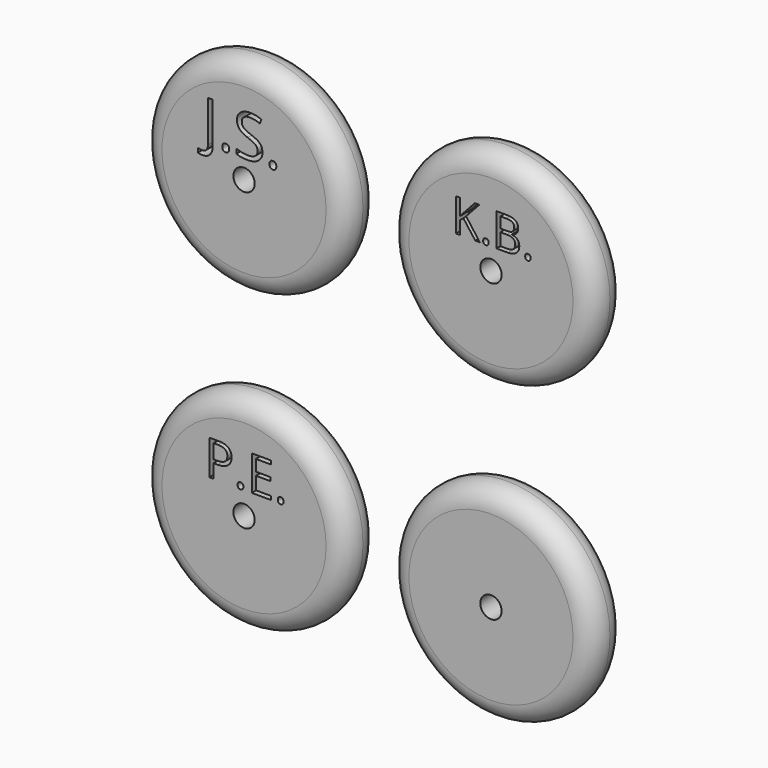
from build123d import *

# Parameters (mm, degrees)
F0_R           = 15.875
F1_DEPTH       = 6.35
F2_R           = 3.17499
F2_2_R         = 3.17499
F2_3_R         = 3.17499
F2_4_R         = 3.17499
F3_R           = 1.651
F4_DEPTH       = 25.4
F5_DEPTH       = 25.4
F6_DEPTH       = 25.4
F7_DEPTH       = 25.4
F8_TEXT_SIZE   = 8.9633877371
F8_TEXT_SIZE_2 = 7.1167148236
F8_TEXT_SIZE_3 = 7.555307678
F9_DEPTH       = 2.54
F10_DEPTH      = 2.54
F12_DEPTH      = 2.54
F11_TEXT_SIZE  = 3.4882623063
F13_DEPTH      = 0.508


# Not quite as in the source:
# - a fillet or chamfer is up to 0.001 mm smaller than in the source, because OpenCascade refuses the exact size
# - Text() gives the source's letters only with a copy of the font that has no kerning and outlines rounded to 1/6400 em; it was checked with that copy


with BuildPart() as f1:
    # F0 (on Front) → F1 (new body)
    with BuildSketch(Plane.XZ):
        with Locations((-57.9834368664, 37.8684985699)):
            Circle(F0_R)
    extrude(amount=F1_DEPTH)

    # F2#3 (radius 3.175 in the source; OpenCascade refuses exactly that, so slightly less here)
    f2_3_edges = [f1.edges().sort_by_distance(p)[0] for p in [
        (-73.858437, 0, 37.868499),
        (-73.858437, -6.35, 37.868499),
    ]]
    fillet(f2_3_edges, radius=F2_3_R)

    # F3 (on face) → F4 (cut)
    with BuildSketch(Plane.XZ.offset(6.35)):
        with Locations((-57.9834368664, 37.8684985699)):
            Circle(F3_R)
    extrude(amount=-F4_DEPTH, mode=Mode.SUBTRACT)


with BuildPart() as f1b:
    # F0 (on Front) → F1, piece 2 (new body)
    with BuildSketch(Plane.XZ):
        with Locations((-57.9834368664, -7.9332944006)):
            Circle(F0_R)
    extrude(amount=F1_DEPTH)

    # F2#4 (radius 3.175 in the source; OpenCascade refuses exactly that, so slightly less here)
    f2_4_edges = [f1b.edges().sort_by_distance(p)[0] for p in [
        (-73.858437, 0, -7.933294),
        (-73.858437, -6.35, -7.933294),
    ]]
    fillet(f2_4_edges, radius=F2_4_R)

    # F3 (on face) → F6 (cut)
    with BuildSketch(Plane.XZ.offset(6.35)):
        with Locations((-57.9834368664, -7.9332944006)):
            Circle(F3_R)
    extrude(amount=-F6_DEPTH, mode=Mode.SUBTRACT)


with BuildPart() as f1c:
    # F0 (on Front) → F1, piece 3 (new body)
    with BuildSketch(Plane.XZ):
        with Locations((-19.7645071894, -7.9332944006)):
            Circle(F0_R)
    extrude(amount=F1_DEPTH)

    # F2 (radius 3.175 in the source; OpenCascade refuses exactly that, so slightly less here)
    f2_edges = [f1c.edges().sort_by_distance(p)[0] for p in [
        (-35.639507, 0, -7.933294),
        (-35.639507, -6.35, -7.933294),
    ]]
    fillet(f2_edges, radius=F2_R)

    # F3 (on face) → F7 (cut)
    with BuildSketch(Plane.XZ.offset(6.35)):
        with Locations((-19.7645071894, -7.9332944006)):
            Circle(F3_R)
    extrude(amount=-F7_DEPTH, mode=Mode.SUBTRACT)


with BuildPart() as f1d:
    # F0 (on Front) → F1, piece 4 (new body)
    with BuildSketch(Plane.XZ):
        with Locations((-19.7645071894, 37.8684985699)):
            Circle(F0_R)
    extrude(amount=F1_DEPTH)

    # F2#2 (radius 3.175 in the source; OpenCascade refuses exactly that, so slightly less here)
    f2_2_edges = [f1d.edges().sort_by_distance(p)[0] for p in [
        (-35.639507, 0, 37.868499),
        (-35.639507, -6.35, 37.868499),
    ]]
    fillet(f2_2_edges, radius=F2_2_R)

    # F3 (on face) → F5 (cut)
    with BuildSketch(Plane.XZ.offset(6.35)):
        with Locations((-19.7645071894, 37.8684985699)):
            Circle(F3_R)
    extrude(amount=-F5_DEPTH, mode=Mode.SUBTRACT)


with BuildPart() as f9_tool:
    # F8 (on face) → F9 (new body)
    with BuildSketch(Plane.XZ.offset(6.35)):
        with Locations((-64.4037676054, 40.8216691305)):
            Text('J.S.', F8_TEXT_SIZE, font='Open Sans', text_align=(TextAlign.LEFT, TextAlign.BOTTOM))
        with Locations((-25.8644149952, 41.2169232358)):
            Text('K.B.', F8_TEXT_SIZE_2, font='Open Sans', text_align=(TextAlign.LEFT, TextAlign.BOTTOM))
        with Locations((-64.0788827856, -4.4081961426)):
            Text('P.E.', F8_TEXT_SIZE_3, font='Open Sans', text_align=(TextAlign.LEFT, TextAlign.BOTTOM))
    extrude(amount=-F9_DEPTH)


with BuildPart() as f1_1:
    add(f1.part)

    # F9: cut by f9_tool
    add(f9_tool.part, mode=Mode.SUBTRACT)

    # F8 (on face) → F10 (cut)
    with BuildSketch(Plane.XZ.offset(6.35)):
        with Locations((-64.4037676054, 40.8216691305)):
            Text('J.S.', F8_TEXT_SIZE, font='Open Sans', text_align=(TextAlign.LEFT, TextAlign.BOTTOM))
        with Locations((-25.8644149952, 41.2169232358)):
            Text('K.B.', F8_TEXT_SIZE_2, font='Open Sans', text_align=(TextAlign.LEFT, TextAlign.BOTTOM))
        with Locations((-64.0788827856, -4.4081961426)):
            Text('P.E.', F8_TEXT_SIZE_3, font='Open Sans', text_align=(TextAlign.LEFT, TextAlign.BOTTOM))
    extrude(amount=-F10_DEPTH, mode=Mode.SUBTRACT)

    # F8 (on face) → F12 (cut)
    with BuildSketch(Plane.XZ.offset(6.35)):
        with Locations((-64.4037676054, 40.8216691305)):
            Text('J.S.', F8_TEXT_SIZE, font='Open Sans', text_align=(TextAlign.LEFT, TextAlign.BOTTOM))
        with Locations((-25.8644149952, 41.2169232358)):
            Text('K.B.', F8_TEXT_SIZE_2, font='Open Sans', text_align=(TextAlign.LEFT, TextAlign.BOTTOM))
        with Locations((-64.0788827856, -4.4081961426)):
            Text('P.E.', F8_TEXT_SIZE_3, font='Open Sans', text_align=(TextAlign.LEFT, TextAlign.BOTTOM))
    extrude(amount=-F12_DEPTH, mode=Mode.SUBTRACT)

    # F11 (on face) → F13 (cut)
    with BuildSketch(Plane.XZ.offset(6.35)):
        with Locations((0.3075196168, 0.3409849917)):
            Text('VROOM', F11_TEXT_SIZE, font='Open Sans', text_align=(TextAlign.LEFT, TextAlign.BOTTOM))
    extrude(amount=-F13_DEPTH, mode=Mode.SUBTRACT)


with BuildPart() as f1b_1:
    add(f1b.part)

    # F9: cut by f9_tool
    add(f9_tool.part, mode=Mode.SUBTRACT)


with BuildPart() as f1d_1:
    add(f1d.part)

    # F9: cut by f9_tool
    add(f9_tool.part, mode=Mode.SUBTRACT)


solid = Compound([f1c.part, f1_1.part, f1b_1.part, f1d_1.part])
